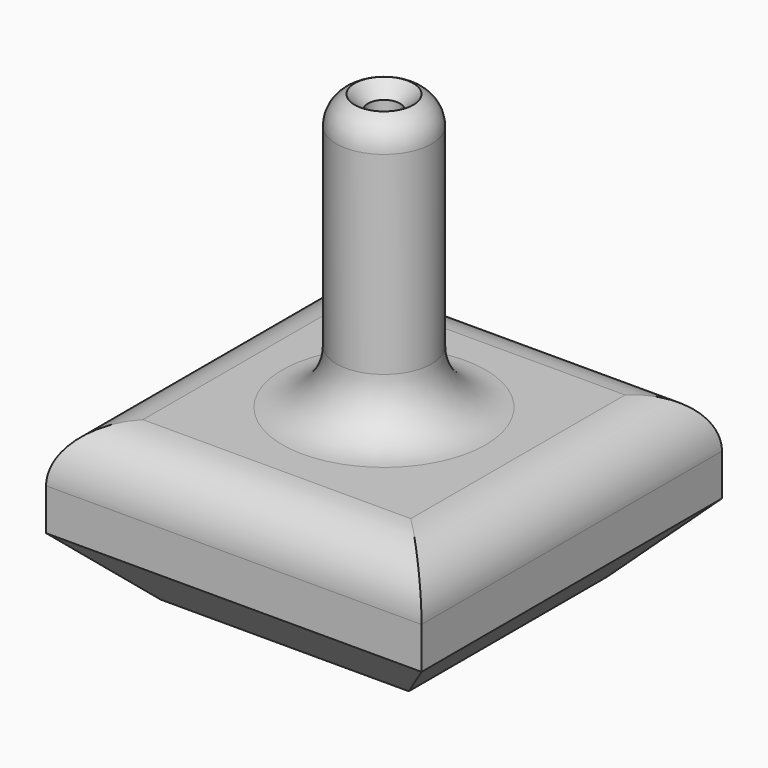
from build123d import *

# Parameters (mm, degrees)
F0_W     = 117.9269552231
F0_H     = 117.9269552231
F0_R     = 15.0136724475
F0_R_2   = 5.0045574825
F1_DEPTH = 50
F2_DEPTH = 137.4
F3_R     = 9.6568542495
F5_R     = 16.8994949366
F6_SIZE  = 20


# Not quite as in the source:
# - a fillet or chamfer that OpenCascade refuses, or shapes differently, is made with other operations: its cross-section is extruded or revolved along the edge and cut away or added


with BuildPart() as f1:
    # F0 (on Top) → F1 (new body)
    with BuildSketch(Plane.XY):
        Rectangle(F0_W, F0_H)
        Circle(F0_R, mode=Mode.SUBTRACT)
        Circle(F0_R)
        Circle(F0_R_2, mode=Mode.SUBTRACT)
    extrude(amount=F1_DEPTH)

    # F0 (on Top) → F2 (join)
    with BuildSketch(Plane.XY):
        Circle(F0_R)
        Circle(F0_R_2, mode=Mode.SUBTRACT)
    extrude(amount=F2_DEPTH)

    # F3
    f3_edges = [f1.edges().sort_by_distance(p)[0] for p in [
        (-15.013672, 0, 137.4),
    ]]
    fillet(f3_edges, radius=F3_R)

    # F4: chamfer of 5 on 1 edges, made by hand

    # F4_s1 → F4_t2 (revolve, cut)
    with BuildSketch(Plane.XZ):
        Polygon((10.0045574825, 137.4), (5.0045574825, 132.4), (5.0045574825, 137.4), align=None)
    revolve(axis=Axis((0, 0, 137.4), (0, 0, 1)), mode=Mode.SUBTRACT)

    # F5
    f5_edges = [f1.edges().sort_by_distance(p)[0] for p in [
        (58.963478, 0, 50),
        (0, -58.963478, 50),
        (0, 58.963478, 50),
        (-58.963478, 0, 50),
        (-15.013672, 0, 50),
    ]]
    fillet(f5_edges, radius=F5_R)

    # F6
    f6_edges = [f1.edges().sort_by_distance(p)[0] for p in [
        (-58.963478, 0, 0),
        (0, 58.963478, 0),
        (58.963478, 0, 0),
        (0, -58.963478, 0),
        (-5.004557, 0, 0),
    ]]
    chamfer(f6_edges, length=F6_SIZE)


solid = f1.part
